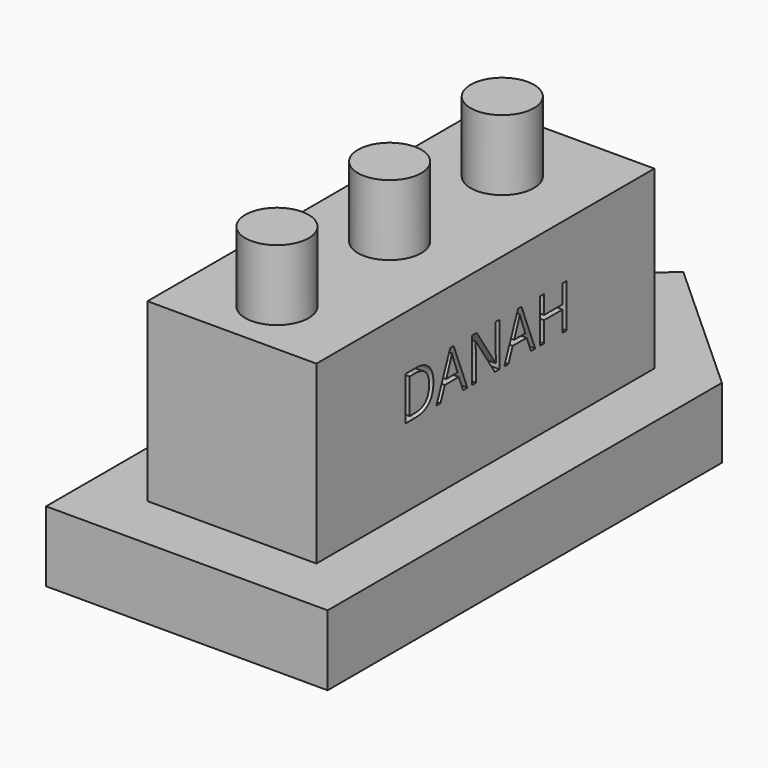
from build123d import *

# Parameters (mm, degrees)
F1_DEPTH     = 10
F2_W         = 24
F2_H         = 60
F3_DEPTH     = 25
F4_R         = 4.5
F5_DEPTH     = 10
F6_TEXT_SIZE = 8.6866036285
F7_DEPTH     = 5


# Not quite as in the source:
# - Text() gives the source's letters only with a copy of the font that has no kerning and outlines rounded to 1/6400 em; it was checked with that copy


with BuildPart() as f1:
    # F0 (on Top) → F1 (new body)
    with BuildSketch(Plane.XY):
        Polygon((0, 41.5285773406), (-20, 23.3902201933), (-20, -46.6097798067), (20, -46.6097798067), (20, 23.3902201933), align=None)
    extrude(amount=F1_DEPTH)

    # F2 (on face) → F3 (join)
    with BuildSketch(Plane.XY.offset(10)):
        with Locations((0, -8.6097798067)):
            Rectangle(F2_W, F2_H)
    extrude(amount=F3_DEPTH)

    # F4 (on face) → F5 (join)
    with BuildSketch(Plane.XY.offset(35)):
        with Locations((0, 9.3902201933)):
            Circle(F4_R)
        with Locations((0, -10.6097798067)):
            Circle(F4_R)
        with Locations((0, -30.6097798067)):
            Circle(F4_R)
    extrude(amount=F5_DEPTH)

    # F6 (on face) → F7 (cut)
    with BuildSketch(Plane.YZ.offset(12)):
        with Locations((-23.6383514037, 21.0835720063)):
            Text('DANAH', F6_TEXT_SIZE, font='Open Sans', text_align=(TextAlign.LEFT, TextAlign.BOTTOM))
    extrude(amount=-F7_DEPTH, mode=Mode.SUBTRACT)


solid = f1.part
